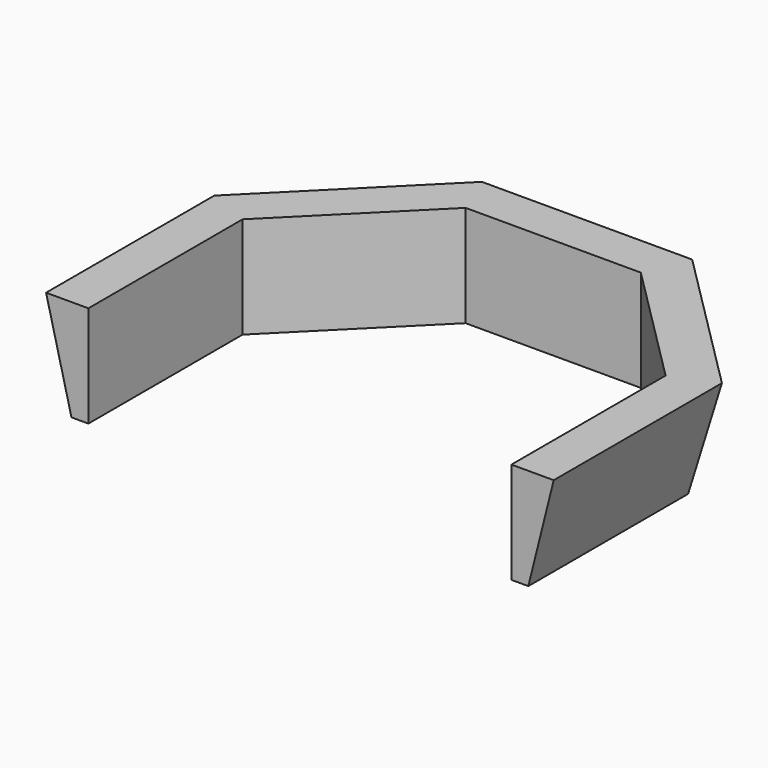
from build123d import *

# Parameters (mm, degrees)
F1_DEPTH = 12
F2_SIZE2 = 11.99999
F2_SIZE  = 2.99999


# Not quite as in the source:
# - a fillet or chamfer is up to 0.001 mm smaller than in the source, because OpenCascade refuses the exact size


with BuildPart() as f1:
    # F0 (on Top) → F1 (new body)
    with BuildSketch(Plane.XY):
        Polygon((12.4264068712, 30), (-12.4264068712, 30), (-30, 12.4264068712), (-30, -12.4264068712), (-25, -12.4264068712), (-25, 10.3553390593), (-10.3553390593, 25), (10.3553390593, 25), (25, 10.3553390593), (25, -12.4264068712), (30, -12.4264068712), (30, 12.4264068712), align=None)
    extrude(amount=F1_DEPTH)

    # F2 (size 3 and 12 in the source; OpenCascade refuses exactly that, so slightly less here)
    f2_edges = [f1.edges().sort_by_distance(p)[0] for p in [
        (-30, 0, 0),
        (-21.213203, 21.213203, 0),
        (0, 30, 0),
        (21.213203, 21.213203, 0),
        (30, 0, 0),
    ]]
    f2_side = f1.faces().sort_by_distance((0, 29.265153, 0))[0]
    chamfer(f2_edges, length=F2_SIZE, length2=F2_SIZE2, reference=f2_side)


solid = f1.part
